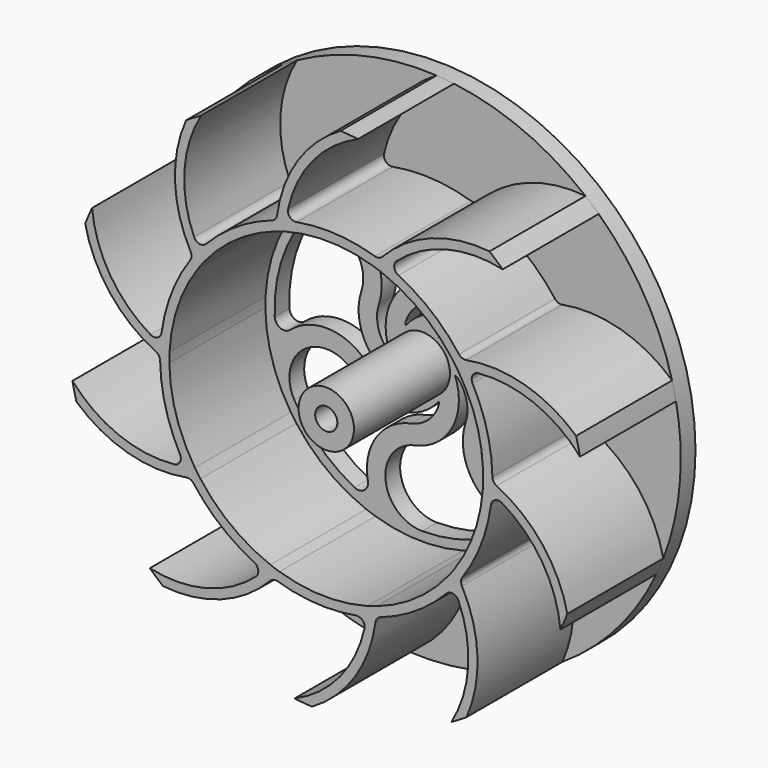
from build123d import *

# Parameters (mm, degrees)
F0_R     = 88.9
F1_DEPTH = 6.35
F2_R     = 57.15
F2_R_2   = 53.975
F3_DEPTH = 41.275
F5_DEPTH = 41.275
F6_R     = 9.525
F6_R_2   = 3.81
F7_DEPTH = 41.275
F8_R     = 3.81
F9_DEPTH = 25.4
F10_R    = 2.54


with BuildPart() as f1:
    # F0 (on Front) → F1 (new body)
    with BuildSketch(Plane.XZ):
        Circle(F0_R)
    extrude(amount=F1_DEPTH)

    # F2 (on face) → F3 (join)
    with BuildSketch(Plane.XZ.offset(6.35)):
        Circle(F2_R)
        Circle(F2_R_2, mode=Mode.SUBTRACT)
    extrude(amount=F3_DEPTH)

    # F4 (on face) → F5 (join, through all)
    with BuildSketch(Plane.XZ.offset(6.35)):
        with BuildLine():
            ThreePointArc((53.9069410952, -2.7096728137), (72.2551452316, -16.3352447412), (80.5410246247, -37.6344702686))
            ThreePointArc((80.5410246247, -37.6344702686), (81.7707619042, -34.8819795541), (82.9064652139, -32.0893755897))
            ThreePointArc((82.9064652139, -32.0893755897), (72.7373983183, -11.9238182989), (53.9711869017, 0.6415679441))
            ThreePointArc((53.9711869017, 0.6415679441), (53.9650843479, -1.0345512645), (53.9069410952, -2.7096728137))
        make_face()
        with BuildLine():
            ThreePointArc((45.2043371792, 29.4935336165), (68.0572563749, 29.2550181665), (87.2800442675, 16.8939004574))
            ThreePointArc((87.2800442675, 16.8939004574), (86.6570491761, 19.8435336593), (85.9344010285, 22.7703473815))
            ThreePointArc((85.9344010285, 22.7703473815), (65.8544359133, 33.10739838), (43.2865032341, 32.2425070794))
            ThreePointArc((43.2865032341, 32.2425070794), (44.2667643164, 30.8829111639), (45.2043371792, 29.4935336165))
        make_face()
        with BuildLine():
            ThreePointArc((19.2352128997, 50.4312126535), (37.863808764, 63.6708584761), (60.6810535397, 64.9693754112))
            ThreePointArc((60.6810535397, 64.9693754112), (58.4432890276, 66.9894914717), (56.1383164531, 68.9325715886))
            ThreePointArc((56.1383164531, 68.9325715886), (33.8173172993, 65.4927141568), (16.0678465853, 51.5279043928))
            ThreePointArc((16.0678465853, 51.5279043928), (17.6600448879, 51.0041511993), (19.2352128997, 50.4312126535))
        make_face()
        with BuildLine():
            ThreePointArc((-14.0811089267, 52.1058825508), (-6.7923268512, 73.7665949407), (10.9039628328, 88.2287571857))
            ThreePointArc((10.9039628328, 88.2287571857), (7.9061788848, 88.547740431), (4.8993030638, 88.7648963808))
            ThreePointArc((4.8993030638, 88.7648963808), (-11.1368671147, 72.8620391412), (-17.2881813331, 51.1313935972))
            ThreePointArc((-17.2881813331, 51.1313935972), (-15.6922114449, 51.6435390438), (-14.0811089267, 52.1058825508))
        make_face()
        with BuildLine():
            ThreePointArc((-42.0189257424, 33.8778763274), (-48.854024472, 55.6859993723), (-43.0380710641, 77.7877525005))
            ThreePointArc((-43.0380710641, 77.7877525005), (-45.6508228708, 76.2837621727), (-48.2110775747, 74.6920477634))
            ThreePointArc((-48.2110775747, 74.6920477634), (-51.837146819, 52.4005416633), (-44.0407115859, 31.2044283397))
            ThreePointArc((-44.0407115859, 31.2044283397), (-43.0505763644, 32.5568502729), (-42.0189257424, 33.8778763274))
        make_face()
        with BuildLine():
            ThreePointArc((-53.9069410952, 2.7096728137), (-72.2551452316, 16.3352447412), (-80.5410246247, 37.6344702686))
            ThreePointArc((-80.5410246247, 37.6344702686), (-81.7707619042, 34.8819795541), (-82.9064652139, 32.0893755897))
            ThreePointArc((-82.9064652139, 32.0893755897), (-72.7373983183, 11.9238182989), (-53.9711869017, -0.6415679441))
            ThreePointArc((-53.9711869017, -0.6415679441), (-53.9650843479, 1.0345512645), (-53.9069410952, 2.7096728137))
        make_face()
        with BuildLine():
            ThreePointArc((-45.2043371792, -29.4935336165), (-68.0572563749, -29.2550181665), (-87.2800442675, -16.8939004574))
            ThreePointArc((-87.2800442675, -16.8939004574), (-86.6570491761, -19.8435336593), (-85.9344010285, -22.7703473815))
            ThreePointArc((-85.9344010285, -22.7703473815), (-65.8544359133, -33.10739838), (-43.2865032341, -32.2425070794))
            ThreePointArc((-43.2865032341, -32.2425070794), (-44.2667643164, -30.8829111639), (-45.2043371792, -29.4935336165))
        make_face()
        with BuildLine():
            ThreePointArc((-19.2352128997, -50.4312126535), (-37.863808764, -63.6708584761), (-60.6810535397, -64.9693754112))
            ThreePointArc((-60.6810535397, -64.9693754112), (-58.4432890276, -66.9894914717), (-56.1383164531, -68.9325715886))
            ThreePointArc((-56.1383164531, -68.9325715886), (-33.8173172993, -65.4927141568), (-16.0678465853, -51.5279043928))
            ThreePointArc((-16.0678465853, -51.5279043928), (-17.6600448879, -51.0041511993), (-19.2352128997, -50.4312126535))
        make_face()
        with BuildLine():
            ThreePointArc((14.0811089267, -52.1058825508), (6.7923268512, -73.7665949407), (-10.9039628328, -88.2287571857))
            ThreePointArc((-10.9039628328, -88.2287571857), (-7.9061788848, -88.547740431), (-4.8993030638, -88.7648963808))
            ThreePointArc((-4.8993030638, -88.7648963808), (11.1368671147, -72.8620391412), (17.2881813331, -51.1313935972))
            ThreePointArc((17.2881813331, -51.1313935972), (15.6922114449, -51.6435390438), (14.0811089267, -52.1058825508))
        make_face()
        with BuildLine():
            ThreePointArc((42.0189257424, -33.8778763274), (48.854024472, -55.6859993723), (43.0380710641, -77.7877525005))
            ThreePointArc((43.0380710641, -77.7877525005), (45.6508228708, -76.2837621727), (48.2110775747, -74.6920477634))
            ThreePointArc((48.2110775747, -74.6920477634), (51.837146819, -52.4005416633), (44.0407115859, -31.2044283397))
            ThreePointArc((44.0407115859, -31.2044283397), (43.0505763644, -32.5568502729), (42.0189257424, -33.8778763274))
        make_face()
    extrude(amount=F5_DEPTH)

    # F6 (on face) → F7 (join, through all)
    with BuildSketch(Plane.XZ.offset(6.35)):
        Circle(F6_R)
        Circle(F6_R_2, mode=Mode.SUBTRACT)
    extrude(amount=F7_DEPTH)

    # F8 (on face) → F9 (cut)
    with BuildSketch(Plane.XZ.offset(6.35)):
        Circle(F8_R)
        with BuildLine():
            ThreePointArc((18.7012290876, 41.7285714286), (15.8576147996, 27.543553966), (3.8682590056, 19.446875))
            ThreePointArc((3.8682590056, 19.446875), (-2.091465664, 16.4126776534), (-5.6835018732, 10.7715831188))
            ThreePointArc((-5.6835018732, 10.7715831188), (-5.7538490333, 10.2503071963), (-5.6500021555, 9.7346589282))
            ThreePointArc((-5.6500021555, 9.7346589282), (8.7313709485, 16.9640191411), (23.5156008127, 10.5989512885))
            ThreePointArc((23.5156008127, 10.5989512885), (40.4349404037, 8.7570054641), (43.9940905122, 25.4))
            ThreePointArc((43.9940905122, 25.4), (35.0538695993, 36.7677334917), (23.2726406424, 45.1555555556))
            ThreePointArc((23.2726406424, 45.1555555556), (19.9136606493, 44.8737532722), (18.7012290876, 41.7285714286))
        make_face()
        with BuildLine():
            ThreePointArc((-11.2554630068, -0.025715934), (-10.3255860522, 16.0435986218), (2.5788393371, 25.6645833333))
            ThreePointArc((2.5788393371, 25.6645833333), (12.6336810088, 39.3961883222), (0, 50.8))
            ThreePointArc((0, 50.8), (-14.3148564437, 48.7414083198), (-27.4695379119, 42.7324757872))
            ThreePointArc((-27.4695379119, 42.7324757872), (-28.9049799722, 39.6826126407), (-26.787388377, 37.0600251862))
            ThreePointArc((-26.787388377, 37.0600251862), (-15.9246100453, 27.5048742428), (-14.9073582714, 13.0734480673))
            ThreePointArc((-14.9073582714, 13.0734480673), (-15.259528624, 6.3950764305), (-12.1702155565, 0.4637345547))
            ThreePointArc((-12.1702155565, 0.4637345547), (-11.7539509452, 0.1421741658), (-11.2554630068, -0.025715934))
        make_face()
        with BuildLine():
            ThreePointArc((-5.6054608513, -9.7603748622), (-19.0569570007, -0.9204205192), (-20.9367614757, 15.0656320448))
            ThreePointArc((-20.9367614757, 15.0656320448), (-27.8012593949, 30.6391828581), (-43.9940905122, 25.4))
            ThreePointArc((-43.9940905122, 25.4), (-49.368726043, 11.9736748281), (-50.7421785543, -2.4230797683))
            ThreePointArc((-50.7421785543, -2.4230797683), (-48.8186406215, -5.1911406315), (-45.4886174646, -4.6685462424))
            ThreePointArc((-45.4886174646, -4.6685462424), (-31.7822248448, -0.0386797232), (-18.775617277, -6.3734269327))
            ThreePointArc((-18.775617277, -6.3734269327), (-13.1680629599, -10.0176012229), (-6.4867136833, -10.3078485641))
            ThreePointArc((-6.4867136833, -10.3078485641), (-6.0001019119, -10.1081330305), (-5.6054608513, -9.7603748622))
        make_face()
        with BuildLine():
            ThreePointArc((5.6500021555, -9.7346589282), (-8.7313709485, -16.9640191411), (-23.5156008127, -10.5989512885))
            ThreePointArc((-23.5156008127, -10.5989512885), (-40.4349404037, -8.7570054641), (-43.9940905122, -25.4))
            ThreePointArc((-43.9940905122, -25.4), (-35.0538695993, -36.7677334917), (-23.2726406424, -45.1555555556))
            ThreePointArc((-23.2726406424, -45.1555555556), (-19.9136606493, -44.8737532722), (-18.7012290876, -41.7285714286))
            ThreePointArc((-18.7012290876, -41.7285714286), (-15.8576147996, -27.543553966), (-3.8682590056, -19.446875))
            ThreePointArc((-3.8682590056, -19.446875), (2.091465664, -16.4126776534), (5.6835018732, -10.7715831188))
            ThreePointArc((5.6835018732, -10.7715831188), (5.7538490333, -10.2503071963), (5.6500021555, -9.7346589282))
        make_face()
        with BuildLine():
            ThreePointArc((11.2554630068, 0.025715934), (10.3255860522, -16.0435986218), (-2.5788393371, -25.6645833333))
            ThreePointArc((-2.5788393371, -25.6645833333), (-12.6336810088, -39.3961883222), (0, -50.8))
            ThreePointArc((0, -50.8), (14.3148564437, -48.7414083198), (27.4695379119, -42.7324757872))
            ThreePointArc((27.4695379119, -42.7324757872), (28.9049799722, -39.6826126407), (26.787388377, -37.0600251862))
            ThreePointArc((26.787388377, -37.0600251862), (15.9246100453, -27.5048742428), (14.9073582714, -13.0734480673))
            ThreePointArc((14.9073582714, -13.0734480673), (15.259528624, -6.3950764305), (12.1702155565, -0.4637345547))
            ThreePointArc((12.1702155565, -0.4637345547), (11.7539509452, -0.1421741658), (11.2554630068, 0.025715934))
        make_face()
        with BuildLine():
            ThreePointArc((5.6054608513, 9.7603748622), (19.0569570007, 0.9204205192), (20.9367614757, -15.0656320448))
            ThreePointArc((20.9367614757, -15.0656320448), (27.8012593949, -30.6391828581), (43.9940905122, -25.4))
            ThreePointArc((43.9940905122, -25.4), (49.368726043, -11.9736748281), (50.7421785543, 2.4230797683))
            ThreePointArc((50.7421785543, 2.4230797683), (48.8186406215, 5.1911406315), (45.4886174646, 4.6685462424))
            ThreePointArc((45.4886174646, 4.6685462424), (31.7822248448, 0.0386797232), (18.775617277, 6.3734269327))
            ThreePointArc((18.775617277, 6.3734269327), (13.1680629599, 10.0176012229), (6.4867136833, 10.3078485641))
            ThreePointArc((6.4867136833, 10.3078485641), (6.0001019119, 10.1081330305), (5.6054608513, 9.7603748622))
        make_face()
    extrude(amount=-F9_DEPTH, mode=Mode.SUBTRACT)

    # F10
    f10_edges = [f1.edges().sort_by_distance(p)[0] for p in [
        (48.482356, -26.9875, 30.258613),
        (57.146896, -26.9875, -0.595661),
        (57.008616, -26.9875, -4.017481),
        (45.882689, -26.9875, -34.072002),
        (43.759523, -26.9875, -36.759035),
        (17.092855, -26.9875, -54.533997),
        (13.795779, -26.9875, -55.459886),
        (-18.225869, -26.9875, -54.165858),
        (-46.58293, -26.9875, -33.108203),
        (-21.437483, -26.9875, -52.976946),
        (-48.482356, -26.9875, -30.258613),
        (-57.008616, -26.9875, 4.017481),
        (-45.882689, -26.9875, 34.072002),
        (-57.146896, -26.9875, 0.595661),
        (-43.759523, -26.9875, 36.759035),
        (-17.092855, -26.9875, 54.533997),
        (-13.795779, -26.9875, 55.459886),
        (18.225869, -26.9875, 54.165858),
        (21.437483, -26.9875, 52.976946),
        (46.58293, -26.9875, 33.108203),
    ]]
    fillet(f10_edges, radius=F10_R)


solid = f1.part
